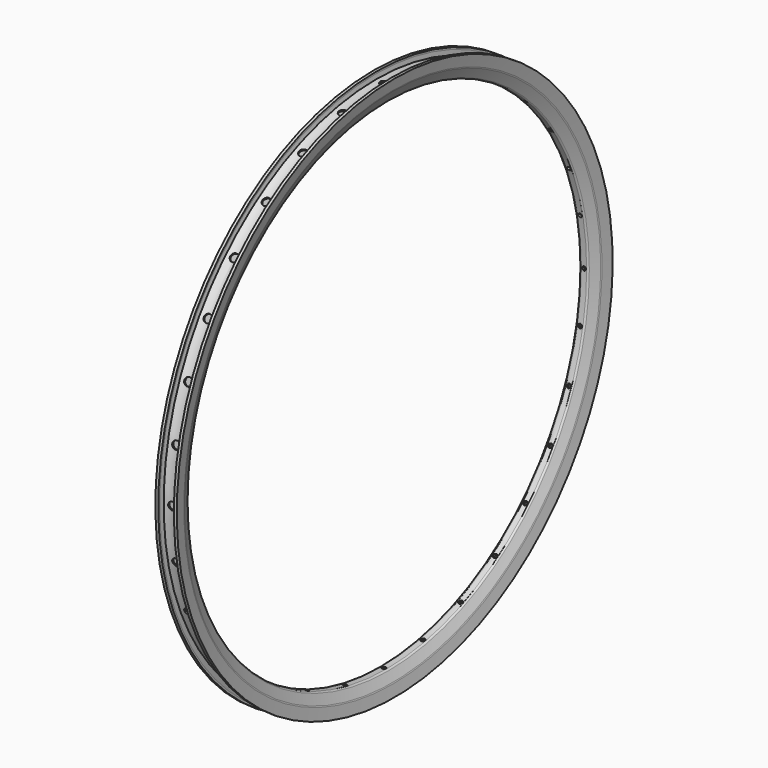
from build123d import *

# Parameters (mm, degrees)
F4_COPIES_COUNT = 32


# Not quite as in the source:
# - a pattern or mirror of a feature is missing from the dataset's text; its kind, count and spacing are read off the source's solid


with BuildPart() as f1:
    # F0 (on Front) → F1 (revolve)
    with BuildSketch(Plane.XZ):
        with BuildLine():
            Line((-8, 279.5), (-11, 279.5))
            Line((-11, 279.5), (-9.1080836513, 268.1485019078))
            ThreePointArc((-9.1080836513, 268.1485019078), (-8.9588318485, 267.512549558), (-8.7279464194, 266.9014821228))
            Line((-8.7279464194, 266.9014821228), (-4.5329064143, 257.6723941114))
            ThreePointArc((-4.5329064143, 257.6723941114), (-3.7949449548, 256.8184513422), (-2.7121734593, 256.5))
            Line((-2.7121734593, 256.5), (2.7121734593, 256.5))
            ThreePointArc((2.7121734593, 256.5), (3.7949449548, 256.8184513422), (4.5329064143, 257.6723941114))
            Line((4.5329064143, 257.6723941114), (8.7279464194, 266.9014821228))
            ThreePointArc((8.7279464194, 266.9014821228), (8.9588318485, 267.512549558), (9.1080836513, 268.1485019078))
            Line((9.1080836513, 268.1485019078), (11, 279.5))
            Line((11, 279.5), (8, 279.5))
            Line((8, 279.5), (8, 277.5))
            Line((8, 277.5), (8.6390791566, 277.5))
            Line((8.6390791566, 277.5), (7.8498060375, 272.7643612858))
            ThreePointArc((7.8498060375, 272.7643612858), (0, 271.5), (-7.8498060375, 272.7643612858))
            Line((-7.8498060375, 272.7643612858), (-8.6390791566, 277.5))
            Line((-8.6390791566, 277.5), (-8, 277.5))
            Line((-8, 277.5), (-8, 279.5))
        make_face()
        with BuildLine():
            Line((7.5732806215, 271.1052087894), (7.1352958036, 268.4772998824))
            ThreePointArc((7.1352958036, 268.4772998824), (7.0457447219, 268.0957284725), (6.9072134645, 267.7290880114))
            Line((6.9072134645, 267.7290880114), (2.7121734593, 258.5))
            Line((2.7121734593, 258.5), (-2.7121734593, 258.5))
            Line((-2.7121734593, 258.5), (-6.9072134645, 267.7290880114))
            ThreePointArc((-6.9072134645, 267.7290880114), (-7.0457447219, 268.0957284725), (-7.1352958036, 268.4772998824))
            Line((-7.1352958036, 268.4772998824), (-7.5732806215, 271.1052087894))
            ThreePointArc((-7.5732806215, 271.1052087894), (0, 270), (7.5732806215, 271.1052087894))
        make_face(mode=Mode.SUBTRACT)
    revolve(axis=Axis((16.0583778866, 0, 0), (1, 0, 0)))

    # F2 (on Front) → F4 (revolve, cut)
    with BuildSketch(Plane.XZ):
        Polygon((-2, 250), (0, 250), (0, 265), (0, 275), (-4, 275), (-4, 265), (-2, 265), align=None)
    f4 = revolve(axis=Axis((0, 0, 270), (0, 0, 1)), mode=Mode.SUBTRACT)

    # F4_copies: F4 ×32 about axis
    f4_copies_axis = Axis((0, 0, 0), (1, 0, 0))
    for i in range(1, F4_COPIES_COUNT):
        add(f4.rotate(f4_copies_axis, i * 360 / F4_COPIES_COUNT), mode=Mode.SUBTRACT)


solid = f1.part
